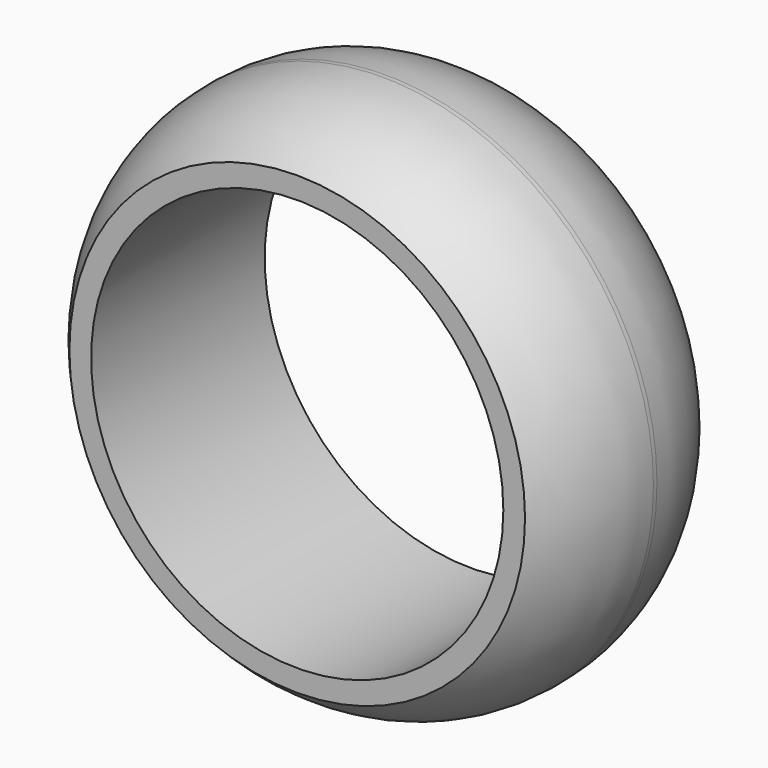
from build123d import *

# Parameters (mm, degrees)
F0_R     = 12.5
F0_R_2   = 10.5
F1_DEPTH = 10
F0_R_3   = 9.5
F3_DEPTH = 10


# Not quite as in the source:
# - a fillet or chamfer that OpenCascade refuses, or shapes differently, is made with other operations: its cross-section is extruded or revolved along the edge and cut away or added


with BuildPart() as f1:
    # F0 (on Front) → F1 (new body)
    with BuildSketch(Plane.XZ):
        Circle(F0_R)
        Circle(F0_R_2, mode=Mode.SUBTRACT)
    extrude(amount=F1_DEPTH)

    # F2: fillet of radius 7 on 3 edges, made by hand

    # F2_s1 → F2_t2 (revolve, cut)
    with BuildSketch(Plane.XY):
        with BuildLine():
            ThreePointArc((12.5, -4.8989794856), (11.9807406984, -2.2532281745), (10.5, 0))
            Line((10.5, 0), (10.6, 0.0979795897))
            ThreePointArc((10.6, 0.0979795897), (11.5, 0.14), (12.5, 0.14))
            Line((12.5, 0.14), (12.64, 0))
            Line((12.64, 0), (12.64, -4.8989794856))
            Line((12.64, -4.8989794856), (12.5, -4.8989794856))
        make_face()
    revolve(axis=Axis((0, 0, 0), (0, -1, 0)), mode=Mode.SUBTRACT)

    # F2_s3 → F2_t4 (revolve, cut)
    with BuildSketch(Plane.XY):
        with BuildLine():
            ThreePointArc((12.5, -5.1010205144), (11.9807406984, -7.7467718255), (10.5, -10))
            Line((10.5, -10), (10.6, -10.0979795897))
            ThreePointArc((10.6, -10.0979795897), (11.5, -10.14), (12.5, -10.14))
            Line((12.5, -10.14), (12.64, -10))
            Line((12.64, -10), (12.64, -5.1010205144))
            Line((12.64, -5.1010205144), (12.5, -5.1010205144))
        make_face()
    revolve(axis=Axis((0, -10, 0), (0, -1, 0)), mode=Mode.SUBTRACT)

    # F0 (on Front) → F3 (join)
    with BuildSketch(Plane.XZ):
        Circle(F0_R_2)
        Circle(F0_R_3, mode=Mode.SUBTRACT)
    extrude(amount=F3_DEPTH)


solid = f1.part
